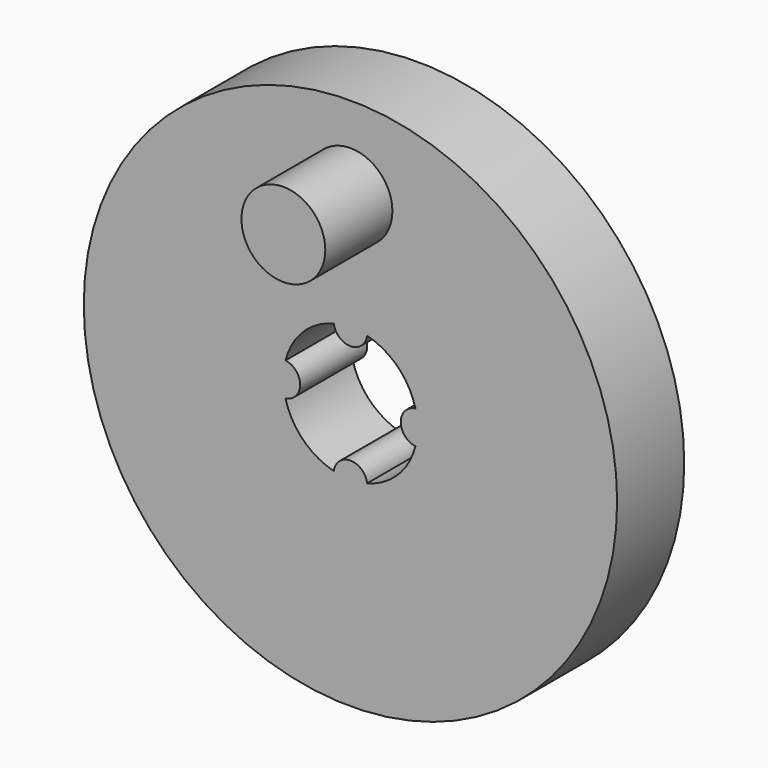
from build123d import *

# Parameters (mm, degrees)
F0_R            = 7.95
F0_R_2          = 2
F1_DEPTH        = 2.5
F2_R            = 1.25
F3_DEPTH        = 2.5
F5_DEPTH        = 2.5
F5_COPIES_COUNT = 4


# Not quite as in the source:
# - a pattern or mirror of a feature is missing from the dataset's text; its kind, count and spacing are read off the source's solid


with BuildPart() as f1:
    # F0 (on Front) → F1 (new body)
    with BuildSketch(Plane.XZ):
        Circle(F0_R)
        Circle(F0_R_2, mode=Mode.SUBTRACT)
    extrude(amount=F1_DEPTH)

    # F2 (on face) → F3 (join)
    with BuildSketch(Plane.XZ.offset(2.5)):
        with Locations((0, 5.45)):
            Circle(F2_R)
    extrude(amount=F3_DEPTH)

    # F4 (on face) → F5 (join, through all)
    with BuildSketch(Plane.XZ.offset(2.5)):
        with BuildLine():
            ThreePointArc((-0.4960783708, 1.9375), (0, 1.5), (0.4960783708, 1.9375))
            ThreePointArc((0.4960783708, 1.9375), (0, 2), (-0.4960783708, 1.9375))
        make_face()
    f5 = extrude(amount=-F5_DEPTH)

    # F5_copies: F5 ×4 about axis
    f5_copies_axis = Axis((0, 0, 0), (0, 1, 0))
    for i in range(1, F5_COPIES_COUNT):
        add(f5.rotate(f5_copies_axis, i * 360 / F5_COPIES_COUNT))


solid = f1.part
